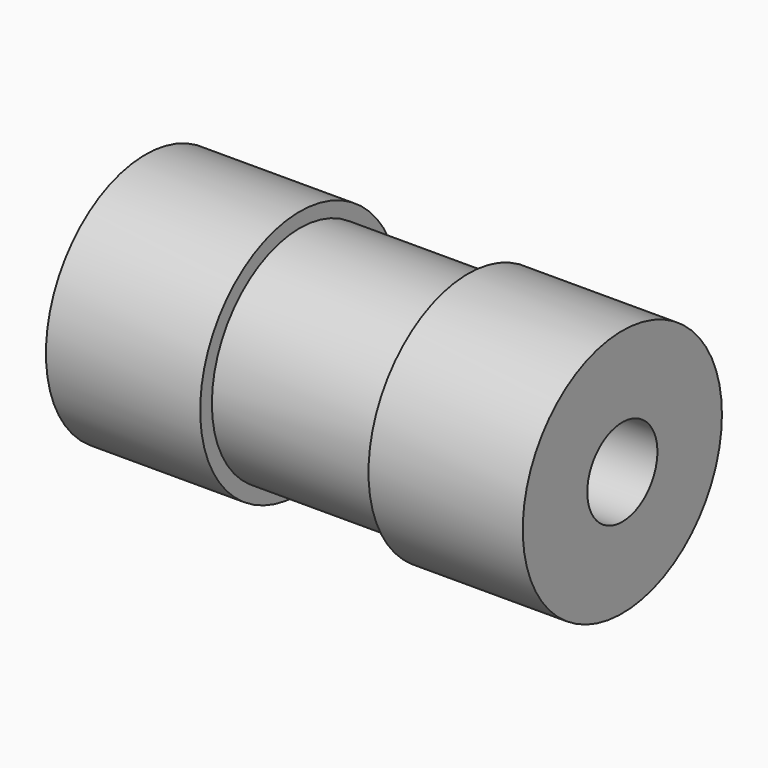
from build123d import *

# Parameters (mm, degrees)
F0_R     = 18.034
F1_DEPTH = 34.544
F2_W     = 24.384
F2_H     = 2.286
F5_D     = 12.7
F5_DEPTH = 22.352
F5_TIP   = 3.8154649308
F7_D     = 15.875
F7_DEPTH = 22.352
F7_TIP   = 4.7693311635


# Not quite as in the source:
# - a length typed as a fraction of an inch, garbled in the dataset ("3 / 203.2 mm" for 3/8 in), is restored


with BuildPart() as f1:
    # F0 (on Right) → F1 (new body, symmetric)
    with BuildSketch(Plane.YZ):
        Circle(F0_R)
    extrude(amount=F1_DEPTH, both=True)

    # F2 (on Front) → F3 (revolve, cut)
    with BuildSketch(Plane.XZ):
        with Locations((0, 17.0634527736)):
            Rectangle(F2_W, F2_H)
    revolve(axis=Axis((6.0458816588, 0, 0), (1, 0, 0)), mode=Mode.SUBTRACT)

    # F5
    with Locations(Plane.YZ.offset(34.544)):
        with Locations((0, 0)):
            Hole(F5_D / 2, depth=F5_DEPTH)
            with Locations((0, 0, -(F5_DEPTH + F5_TIP / 2))):  # 118° drill point
                Cone(0, F5_D / 2, F5_TIP, mode=Mode.SUBTRACT)

    # F7
    with Locations(Plane(origin=(-34.544, 0, 0), x_dir=(0, -1, 0), z_dir=(-1, 0, 0))):
        with Locations((0, 0)):
            Hole(F7_D / 2, depth=F7_DEPTH)
            with Locations((0, 0, -(F7_DEPTH + F7_TIP / 2))):  # 118° drill point
                Cone(0, F7_D / 2, F7_TIP, mode=Mode.SUBTRACT)


solid = f1.part
